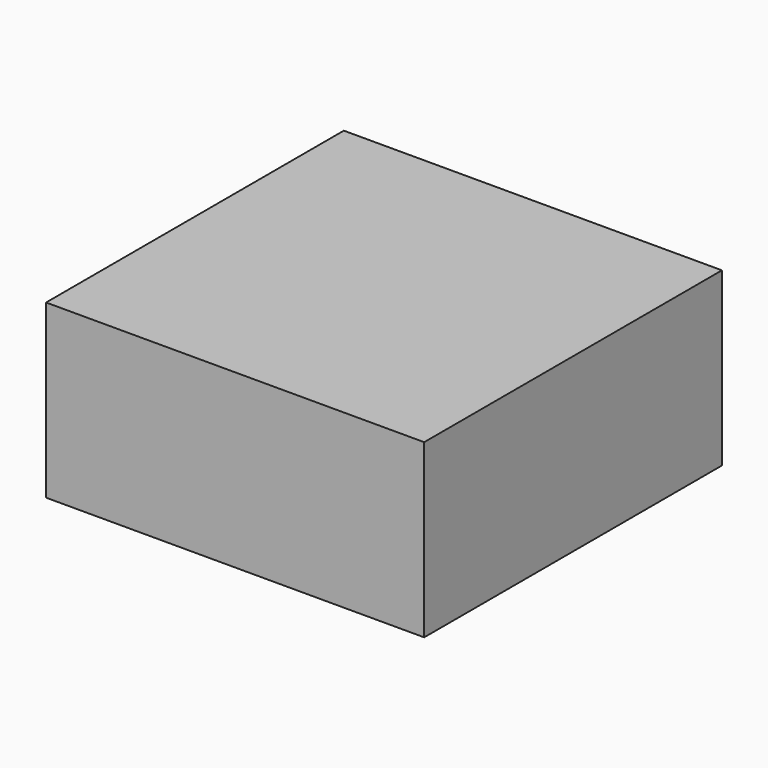
from build123d import *

# Parameters (mm, degrees)
F1_R     = 9.8246353949
F2_DEPTH = 63.5
F0_W     = 69.8630958796
F0_H     = 137.5265717506


# Not quite as in the source:
# - the program builds the solid bodies; features that only make, move or delete a surface that nothing else refers to are left out


with BuildPart() as f2:
    # F1 (on Top) → F2 (new body)
    with BuildSketch(Plane.XY):
        with Locations((54.2640089989, 0)):
            Circle(F1_R)
    extrude(amount=F2_DEPTH)


with BuildPart() as f2b:
    # F0 (on Top) → F2, piece 2 (new body)
    with BuildSketch(Plane.XY):
        with Locations((34.9315479398, 0)):
            Rectangle(F0_W, F0_H)
        with Locations((-34.9315479398, 0)):
            Rectangle(F0_W, F0_H)
    extrude(amount=F2_DEPTH)


solid = Compound([f2.part, f2b.part])
